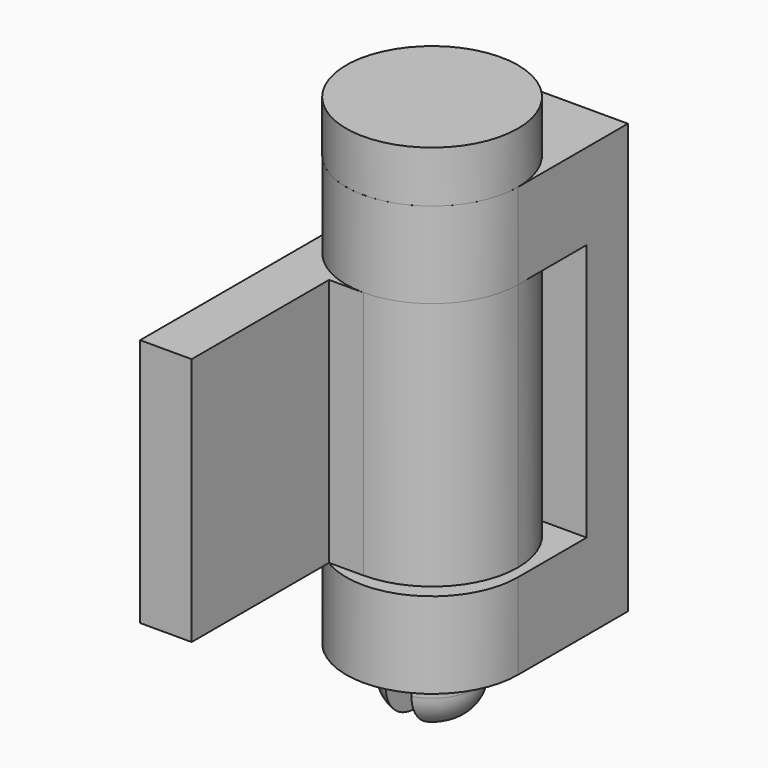
from build123d import *

# Parameters (mm, degrees)
F0_W      = 10
F0_H      = 25
F1_DEPTH  = 3
F2_R      = 2.5
F3_DEPTH  = 5
F4_START  = -20
F3_FACE_R = 2.5
F4_DEPTH  = 5
F6_DEPTH  = 14.5
F7_R      = 2.5
F7_R_2    = 2.3
F8_DEPTH  = 3
F9_DEPTH  = 25.5
F10_R     = 2.55
F11_DEPTH = 3
F12_R     = 2
F13_W     = 1.5
F13_H     = 8
F14_DEPTH = 5


with BuildPart() as f1:
    # F0 (on Front) → F1 (new body)
    with BuildSketch(Plane.XZ):
        with Locations((5, 12.5)):
            Rectangle(F0_W, F0_H)
    extrude(amount=F1_DEPTH)

    # F2 (on face) → F3 (join)
    with BuildSketch(Plane(origin=(0, 0, 0), x_dir=(1, 0, 0), z_dir=(0, 0, -1))):
        with BuildLine():
            ThreePointArc((5, 3), (8.5355339059, 4.4644660941), (10, 8))
            ThreePointArc((10, 8), (5, 13), (0, 8))
            ThreePointArc((0, 8), (1.4644660941, 4.4644660941), (5, 3))
        make_face()
        with Locations((5, 8)):
            Circle(F2_R, mode=Mode.SUBTRACT)
        with BuildLine():
            ThreePointArc((5, 3), (1.4644660941, 4.4644660941), (0, 8))
            Line((0, 8), (0, 3))
            Line((0, 3), (5, 3))
        make_face()
        with BuildLine():
            Line((10, 3), (10, 8))
            ThreePointArc((10, 8), (8.5355339059, 4.4644660941), (5, 3))
            Line((5, 3), (10, 3))
        make_face()
    extrude(amount=-F3_DEPTH)

    # F3_face (on face) → F4 (join)
    with BuildSketch(Plane(origin=(5, -5.6246622599, 0), x_dir=(1, 0, 0), z_dir=(0, 0, -1)).offset(F4_START)):
        with BuildLine():
            Line((-5, 2.3753377401), (-5, -5.6246622599))
            Line((-5, -5.6246622599), (5, -5.6246622599))
            Line((5, -5.6246622599), (5, 2.3753377401))
            ThreePointArc((5, 2.3753377401), (0, 7.3753377401), (-5, 2.3753377401))
        make_face()
        with Locations((0, 2.3753377401)):
            Circle(F3_FACE_R, mode=Mode.SUBTRACT)
    extrude(amount=-F4_DEPTH)


with BuildPart() as f6:
    # F5 (on face) → F6 (new body)
    with BuildSketch(Plane(origin=(0, 0, 20), x_dir=(1, 0, 0), z_dir=(0, 0, -1))):
        with BuildLine():
            ThreePointArc((0, 8), (0.8166998673, 10.7386127875), (3, 12.582575695))
            Line((3, 12.582575695), (3, 13))
            Line((3, 13), (3, 23))
            Line((3, 23), (0, 23))
            Line((0, 23), (0, 8))
        make_face()
        with BuildLine():
            Line((3, 9.5), (3, 12.582575695))
            ThreePointArc((3, 12.582575695), (0.8166998673, 10.7386127875), (0, 8))
            ThreePointArc((0, 8), (0.8166998673, 5.2613872125), (3, 3.417424305))
            Line((3, 3.417424305), (3, 6.5))
            ThreePointArc((3, 6.5), (2.5, 8), (3, 9.5))
        make_face()
        with BuildLine():
            Line((3, 3), (3, 3.417424305))
            ThreePointArc((3, 3.417424305), (0.8166998673, 5.2613872125), (0, 8))
            Line((0, 8), (0, 3))
            Line((0, 3), (3, 3))
        make_face()
        with BuildLine():
            ThreePointArc((5, 3), (8.5355339059, 4.4644660941), (10, 8))
            ThreePointArc((10, 8), (8.5355339059, 11.5355339059), (5, 13))
            ThreePointArc((5, 13), (3.9784517816, 12.8945315647), (3, 12.582575695))
            Line((3, 12.582575695), (3, 9.5))
            ThreePointArc((3, 9.5), (5.790569415, 10.3717082451), (7.5, 8))
            ThreePointArc((7.5, 8), (5.790569415, 5.6282917549), (3, 6.5))
            Line((3, 6.5), (3, 3.417424305))
            ThreePointArc((3, 3.417424305), (3.9784517816, 3.1054684353), (5, 3))
        make_face()
        with BuildLine():
            Line((3, 3), (5, 3))
            ThreePointArc((5, 3), (3.9784517816, 3.1054684353), (3, 3.417424305))
            Line((3, 3.417424305), (3, 3))
        make_face()
        with BuildLine():
            ThreePointArc((3, 12.582575695), (3.9784517816, 12.8945315647), (5, 13))
            Line((5, 13), (3, 13))
            Line((3, 13), (3, 12.582575695))
        make_face()
    extrude(amount=F6_DEPTH)


with BuildPart() as f8:
    # F7 (on face) → F8 (new body)
    with BuildSketch(Plane.XY.offset(25)):
        with BuildLine():
            ThreePointArc((0, -8), (5, -13), (10, -8))
            ThreePointArc((10, -8), (5, -3), (0, -8))
        make_face()
        with Locations((5, -8)):
            Circle(F7_R, mode=Mode.SUBTRACT)
        with Locations((5, -8)):
            Circle(F7_R)
        with Locations((5, -8)):
            Circle(F7_R_2, mode=Mode.SUBTRACT)
        with Locations((5, -8)):
            Circle(F7_R_2)
    extrude(amount=F8_DEPTH)

    # F7 (on face) → F9 (join)
    with BuildSketch(Plane.XY.offset(25)):
        with Locations((5, -8)):
            Circle(F7_R_2)
    extrude(amount=-F9_DEPTH)

    # F10 (on face) → F11 (join)
    with BuildSketch(Plane(origin=(0, 0, -0.5), x_dir=(1, 0, 0), z_dir=(0, 0, -1))):
        with Locations((5, 8)):
            Circle(F10_R)
    extrude(amount=F11_DEPTH)

    # F12
    f12_edges = [f8.edges().sort_by_distance(p)[0] for p in [
        (2.45, -8, -3.5),
    ]]
    fillet(f12_edges, radius=F12_R)

    # F13 (on face) → F14 (cut)
    with BuildSketch(Plane(origin=(0, 0, -3.5), x_dir=(1, 0, 0), z_dir=(0, 0, -1))):
        with Locations((5, 8)):
            Rectangle(F13_W, F13_H)
    extrude(amount=-F14_DEPTH, mode=Mode.SUBTRACT)


solid = Compound([f1.part, f6.part, f8.part])
